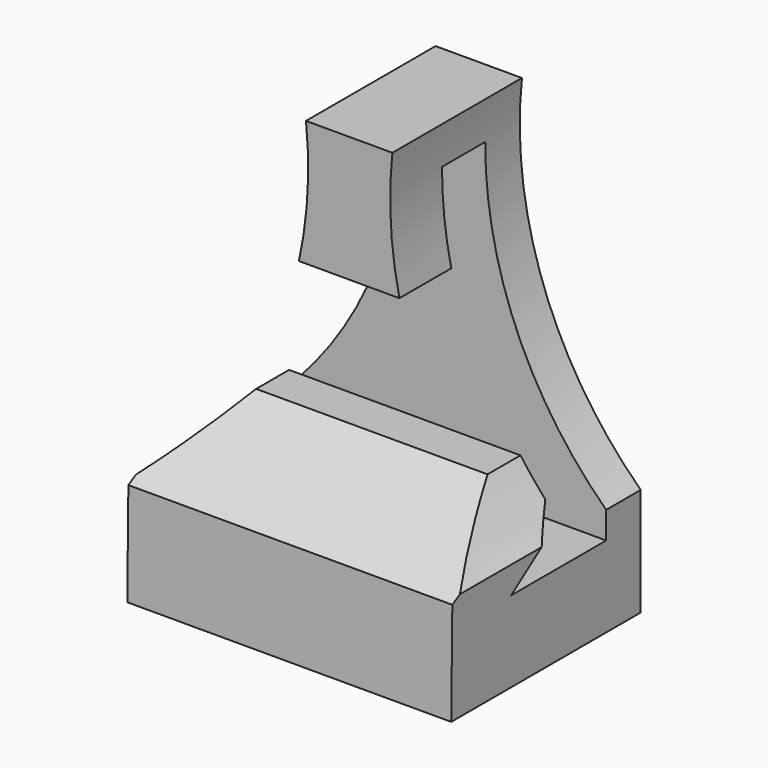
from build123d import *

# Parameters (mm, degrees)
F1_DEPTH = 60
F3_DEPTH = 43.8751131995


# Not quite as in the source:
# - a pattern or mirror of a feature is missing from the dataset's text; its kind, count and spacing are read off the source's solid


with BuildPart() as f1:
    # F0 (on Right) → F1 (new body)
    with BuildSketch(Plane.YZ):
        Polygon((-43.8741131995, 0), (0, 0), (0, 80), (-30, 80), (-30, 56.7161887884), (-18, 56.7161887884), (-18, 72.701357305), (-8, 72.701357305), (-8, 15), (-30, 15), (-17.1229156852, 24.1054718941), (-17.1229156852, 29.8044607043), (-24.7526019812, 29.8044607043), (-43.619140311, 18.9982891026), align=None)
    extrude(amount=F1_DEPTH)

    # F2 (on face) → F3 (cut, through all)
    with BuildSketch(Plane(origin=(0, 0, 0), x_dir=(-1, 0, 0), z_dir=(0, 1, 0))):
        with BuildLine():
            Line((-60, 80), (-60, 20))
            ThreePointArc((-60, 20), (-42.0220624026, 47.4414228809), (-38, 80))
            Line((-38, 80), (-60, 80))
        make_face()
    f3 = extrude(amount=-F3_DEPTH, mode=Mode.SUBTRACT)

    # F3_copies: F3 across plane
    add(f3.mirror(Plane(origin=(30, 0, 0), x_dir=(0, 0, -1), z_dir=(-1, 0, 0))), mode=Mode.SUBTRACT)


solid = f1.part
